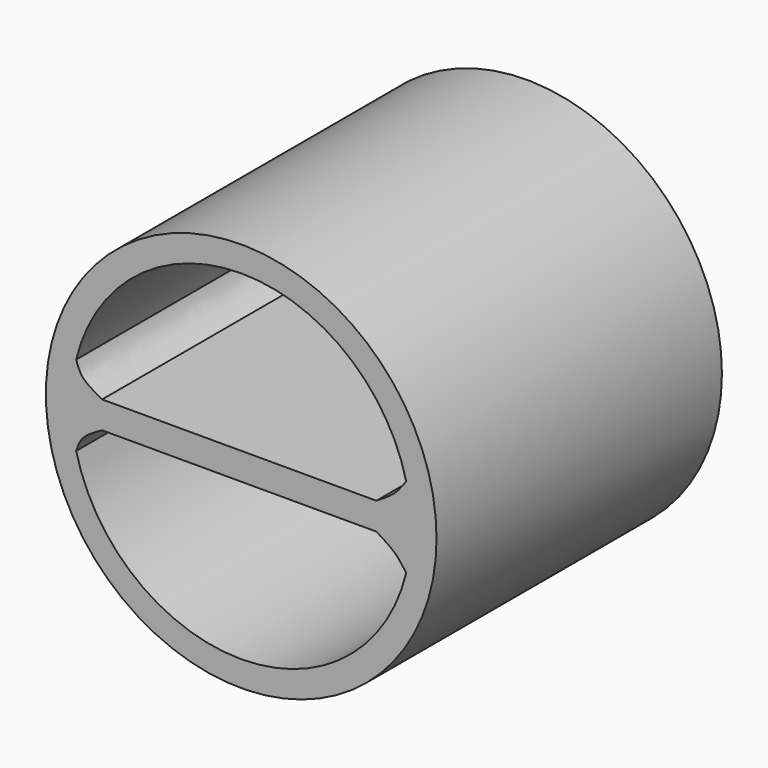
from build123d import *

# Parameters (mm, degrees)
F0_R     = 73.025
F1_DEPTH = 133.35
F2_DEPTH = 25.4


with BuildPart() as f1:
    # F0 (on Front) → F1 (new body)
    with BuildSketch(Plane.XZ):
        Circle(F0_R)
        with BuildLine():
            ThreePointArc((63.2964738354, 5.08), (63.4490980572, 2.5420377112), (63.5, 0))
            ThreePointArc((63.5, 0), (63.4490980572, -2.5420377112), (63.2964738354, -5.08))
            ThreePointArc((63.2964738354, -5.08), (62.6939870382, -10.0853353566), (61.696322928, -15.0271000916))
            ThreePointArc((61.696322928, -15.0271000916), (0, -63.5), (-61.696322928, -15.0271000916))
            ThreePointArc((-61.696322928, -15.0271000916), (-62.6939870382, -10.0853353566), (-63.2964738354, -5.08))
            ThreePointArc((-63.2964738354, -5.08), (-63.5, 0), (-63.2964738354, 5.08))
            ThreePointArc((-63.2964738354, 5.08), (-62.6939870382, 10.0853353566), (-61.696322928, 15.0271000916))
            ThreePointArc((-61.696322928, 15.0271000916), (0, 63.5), (61.696322928, 15.0271000916))
            ThreePointArc((61.696322928, 15.0271000916), (62.6939870382, 10.0853353566), (63.2964738354, 5.08))
        make_face(mode=Mode.SUBTRACT)
        with BuildLine():
            ThreePointArc((63.2964738354, -5.08), (63.4490980572, -2.5420377112), (63.5, 0))
            ThreePointArc((63.5, 0), (63.4490980572, 2.5420377112), (63.2964738354, 5.08))
            Line((63.2964738354, 5.08), (50.5231209099, 5.08))
            Line((50.5231209099, 5.08), (-8.6646769196, 5.08))
            Line((-8.6646769196, 5.08), (-51.9901923835, 5.08))
            Line((-51.9901923835, 5.08), (-63.2964738354, 5.08))
            ThreePointArc((-63.2964738354, 5.08), (-63.5, 0), (-63.2964738354, -5.08))
            Line((-63.2964738354, -5.08), (-51.9901923835, -5.08))
            Line((-51.9901923835, -5.08), (-8.6646769196, -5.08))
            Line((-8.6646769196, -5.08), (50.5231209099, -5.08))
            Line((50.5231209099, -5.08), (63.2964738354, -5.08))
        make_face()
        with BuildLine():
            Line((50.5231209099, 5.08), (63.2964738354, 5.08))
            ThreePointArc((63.2964738354, 5.08), (62.6939870382, 10.0853353566), (61.696322928, 15.0271000916))
            add(Edge.make_bspline(
                [(61.696322928, 15.0271000916), (60.4599662433, 13.2835631459), (57.8112317295, 9.5482604282), (53.0577875896, 6.6339762092), (50.5231209099, 5.08)],
                knots=[0, 0, 0, 0, 0.4667725958, 1, 1, 1, 1], degree=3))
        make_face()
        with BuildLine():
            ThreePointArc((61.696322928, -15.0271000916), (62.6939870382, -10.0853353566), (63.2964738354, -5.08))
            Line((63.2964738354, -5.08), (50.5231209099, -5.08))
            add(Edge.make_bspline(
                [(61.696322928, -15.0271000916), (60.4599662433, -13.2835631459), (57.8112317295, -9.5482604282), (53.0577875896, -6.6339762092), (50.5231209099, -5.08)],
                knots=[0, 0, 0, 0, 0.4667725958, 1, 1, 1, 1], degree=3))
        make_face()
        with BuildLine():
            add(Edge.make_bspline(
                [(-61.696322928, 15.0271000916), (-61.1179777584, 13.2619750664), (-59.7584225638, 9.3012859588), (-54.7646458459, 6.5824467775), (-51.9901923835, 5.08)],
                knots=[0, 0, 0, 0, 0.4461018831, 1, 1, 1, 1], degree=3))
            ThreePointArc((-61.696322928, 15.0271000916), (-62.6939870382, 10.0853353566), (-63.2964738354, 5.08))
            Line((-63.2964738354, 5.08), (-51.9901923835, 5.08))
        make_face()
        with BuildLine():
            ThreePointArc((-63.2964738354, -5.08), (-62.6939870382, -10.0853353566), (-61.696322928, -15.0271000916))
            add(Edge.make_bspline(
                [(-61.696322928, -15.0271000916), (-61.1179777584, -13.2619750664), (-59.7584225638, -9.3012859588), (-54.7646458459, -6.5824467775), (-51.9901923835, -5.08)],
                knots=[0, 0, 0, 0, 0.4461018831, 1, 1, 1, 1], degree=3))
            Line((-51.9901923835, -5.08), (-63.2964738354, -5.08))
        make_face()
    extrude(amount=F1_DEPTH)

    # F0 (on Front) → F2 (join)
    with BuildSketch(Plane.XZ):
        with BuildLine():
            add(Edge.make_bspline(
                [(61.696322928, 15.0271000916), (60.4599662433, 13.2835631459), (57.8112317295, 9.5482604282), (53.0577875896, 6.6339762092), (50.5231209099, 5.08)],
                knots=[0, 0, 0, 0, 0.4667725958, 1, 1, 1, 1], degree=3))
            ThreePointArc((61.696322928, 15.0271000916), (0, 63.5), (-61.696322928, 15.0271000916))
            add(Edge.make_bspline(
                [(-61.696322928, 15.0271000916), (-61.1179777584, 13.2619750664), (-59.7584225638, 9.3012859588), (-54.7646458459, 6.5824467775), (-51.9901923835, 5.08)],
                knots=[0, 0, 0, 0, 0.4461018831, 1, 1, 1, 1], degree=3))
            Line((-51.9901923835, 5.08), (-8.6646769196, 5.08))
            Line((-8.6646769196, 5.08), (50.5231209099, 5.08))
        make_face()
        with BuildLine():
            ThreePointArc((-61.696322928, -15.0271000916), (0, -63.5), (61.696322928, -15.0271000916))
            add(Edge.make_bspline(
                [(61.696322928, -15.0271000916), (60.4599662433, -13.2835631459), (57.8112317295, -9.5482604282), (53.0577875896, -6.6339762092), (50.5231209099, -5.08)],
                knots=[0, 0, 0, 0, 0.4667725958, 1, 1, 1, 1], degree=3))
            Line((50.5231209099, -5.08), (-8.6646769196, -5.08))
            Line((-8.6646769196, -5.08), (-51.9901923835, -5.08))
            add(Edge.make_bspline(
                [(-61.696322928, -15.0271000916), (-61.1179777584, -13.2619750664), (-59.7584225638, -9.3012859588), (-54.7646458459, -6.5824467775), (-51.9901923835, -5.08)],
                knots=[0, 0, 0, 0, 0.4461018831, 1, 1, 1, 1], degree=3))
        make_face()
    extrude(amount=F2_DEPTH)


solid = f1.part
